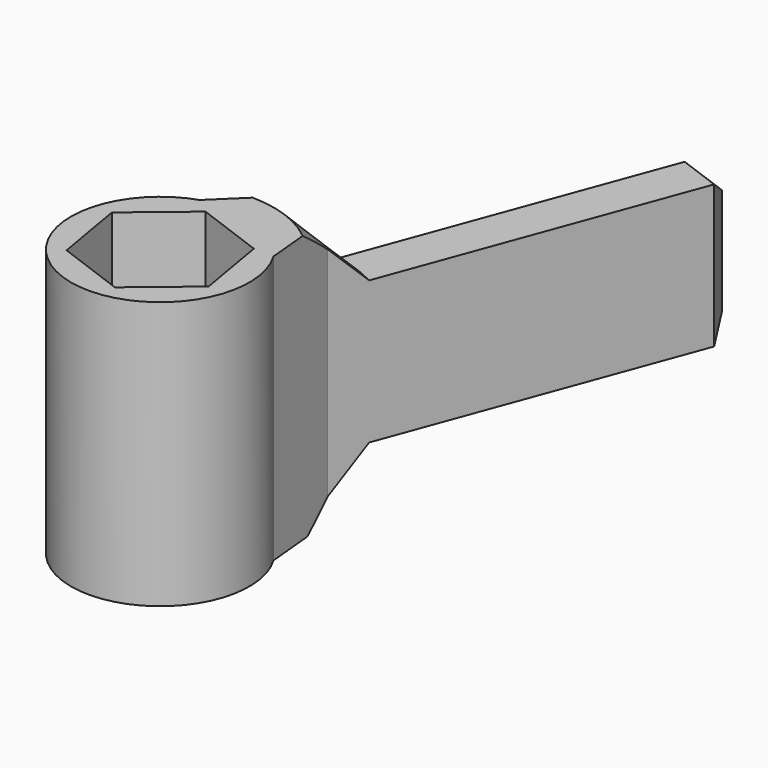
from build123d import *

# Parameters (mm, degrees)
F0_R         = 5
F1_DEPTH     = 15
F2_W         = 2.5
F2_H         = 8
F3_DEPTH     = 25
F4_T1_DEPTH  = 8
F4_T6_ANGLE  = 323.6604372277
F4_T13_ANGLE = 323.6604372277
F4_T21_ANGLE = 323.6604372277
F4_T26_DEPTH = 15.8662197745
F4_T34_ANGLE = 323.6604372277
F4_T39_DEPTH = 15.8662197745
F4_T47_DEPTH = 15.8662197745
F4_T52_ANGLE = 323.6604372277
F4_T60_ANGLE = 323.6604372277
F4_T65_DEPTH = 15.8662197745
F5_SIZE      = 1


# Not quite as in the source:
# - a fillet or chamfer that OpenCascade refuses, or shapes differently, is made with other operations: its cross-section is extruded or revolved along the edge and cut away or added


with BuildPart() as f1:
    # F0 (on Top) → F1 (new body)
    with BuildSketch(Plane.XY):
        Circle(F0_R)
        Polygon((3.1522870356, 2.6203854256), (3.8454638641, -1.4197679401), (0.6931768285, -4.0401533656), (-3.1522870356, -2.6203854256), (-3.8454638641, 1.4197679401), (-0.6931768285, 4.0401533656), align=None, mode=Mode.SUBTRACT)
    extrude(amount=F1_DEPTH)

    # F2 (on face) → F3 (join)
    with BuildSketch(Plane(origin=(1.2295551036, 3.3302693956, 0), x_dir=(0.9381040551, -0.3463535503, 0), z_dir=(-0.3463535503, -0.9381040551, 0))):
        with Locations((0, 7.3666626269)):
            Rectangle(F2_W, F2_H)
    extrude(amount=-F3_DEPTH)

    # F4: chamfer of 5 on 4 edges, made by hand

    # F4_s2 → F4_t1 (join)
    with BuildSketch(Plane.XY.offset(3.3666626269)):
        with BuildLine():
            Line((-1.5797144045, 4.7438910612), (1.5310914666, 7.7560143709))
            Line((1.5310914666, 7.7560143709), (0.5041468464, 4.9745186659))
            ThreePointArc((0.5041468464, 4.9745186659), (-0.631305898, 4.9599851676), (-1.5797144045, 4.7438910612))
        make_face()
        with BuildLine():
            Line((4.2834359399, 2.5791813718), (3.8763516043, 6.8901304951))
            Line((3.8763516043, 6.8901304951), (2.8494069841, 4.1086347901))
            ThreePointArc((2.8494069841, 4.1086347901), (3.702995808, 3.359735413), (4.2834359399, 2.5791813718))
        make_face()
    extrude(amount=F4_T1_DEPTH)


with BuildPart() as f4_tool4:
    # F4_s5 → F4_t6 (revolve)
    with BuildSketch(Plane(origin=(0, 0, 0), x_dir=(0, 0, 1), z_dir=(0.7833222839, -0.6216157974, 0))):
        Polygon((16.3666626269, 5), (11.3666626269, 10), (11.3666626269, 5), align=None)
    revolve(axis=Axis((0, 0, 11.3666626269), (0, 0, -1)), revolution_arc=F4_T6_ANGLE)

    split(bisect_by=Plane.XY.offset(15), keep=Keep.BOTTOM)

    split(bisect_by=Plane(origin=(-1.1726300689, 0.4329419379, 0), x_dir=(0, 0, 1), z_dir=(0.9381040551, -0.3463535503, 0)), keep=Keep.TOP)

    split(bisect_by=Plane(origin=(1.1726300689, -0.4329419379, 0), x_dir=(0, 0, 1), z_dir=(-0.9381040551, 0.3463535503, 0)), keep=Keep.TOP)


with BuildPart() as f1_1:
    add(f1.part)

    # F4_t3: union F4_tool4
    add(f4_tool4.part)


with BuildPart() as f4_tool11:
    # F4_s12 → F4_t13 (revolve)
    with BuildSketch(Plane(origin=(0, 0, 0), x_dir=(0, 0, 1), z_dir=(0.7833222839, -0.6216157974, 0))):
        Polygon((-1.6333373731, 5), (3.3666626269, 10), (3.3666626269, 5), align=None)
    revolve(axis=Axis((0, 0, 3.3666626269), (0, 0, -1)), revolution_arc=F4_T13_ANGLE)

    split(bisect_by=Plane.XY, keep=Keep.TOP)

    split(bisect_by=Plane(origin=(-1.1726300689, 0.4329419379, 0), x_dir=(0, 0, 1), z_dir=(0.9381040551, -0.3463535503, 0)), keep=Keep.TOP)

    split(bisect_by=Plane(origin=(1.1726300689, -0.4329419379, 0), x_dir=(0, 0, 1), z_dir=(-0.9381040551, 0.3463535503, 0)), keep=Keep.TOP)


with BuildPart() as f1_2:
    add(f1_1.part)

    # F4_t10: union F4_tool11
    add(f4_tool11.part)


with BuildPart() as f4_tool19:
    # F4_s20 → F4_t21 (revolve)
    with BuildSketch(Plane(origin=(0, 0, 0), x_dir=(0, 0, 1), z_dir=(0.7833222839, -0.6216157974, 0))):
        Polygon((16.3666626269, 5), (11.3666626269, 10), (11.3666626269, 5), align=None)
    revolve(axis=Axis((0, 0, 11.3666626269), (0, 0, -1)), revolution_arc=F4_T21_ANGLE)

    split(bisect_by=Plane.XY.offset(15), keep=Keep.BOTTOM)

    split(bisect_by=Plane(origin=(-1.1726300689, 0.4329419379, 0), x_dir=(0, 0, 1), z_dir=(-0.9381040551, 0.3463535503, 0)), keep=Keep.TOP)


with BuildPart() as f4_tool24:
    # F4_s25 → F4_t26 (new body)
    with BuildSketch(Plane.XY.offset(19.2328824014)):
        with BuildLine():
            Line((-1.5797144045, 4.7438910612), (1.5310914666, 7.7560143709))
            Line((1.5310914666, 7.7560143709), (0.5041468464, 4.9745186659))
            ThreePointArc((0.5041468464, 4.9745186659), (-0.631305898, 4.9599851676), (-1.5797144045, 4.7438910612))
        make_face()
    extrude(amount=-F4_T26_DEPTH)

    split(bisect_by=Plane.XY.offset(15), keep=Keep.BOTTOM)

    split(bisect_by=Plane.XY.offset(11.3666626269), keep=Keep.TOP)


with BuildPart() as f4_tool19_1:
    add(f4_tool19.part)

    # F4_t29: intersect F4_tool24
    add(f4_tool24.part, mode=Mode.INTERSECT)


with BuildPart() as f1_3:
    add(f1_2.part)

    # F4_t17: union F4_tool19
    add(f4_tool19_1.part)


with BuildPart() as f4_tool32:
    # F4_s33 → F4_t34 (revolve)
    with BuildSketch(Plane(origin=(0, 0, 0), x_dir=(0, 0, 1), z_dir=(0.7833222839, -0.6216157974, 0))):
        Polygon((16.3666626269, 5), (11.3666626269, 10), (11.3666626269, 5), align=None)
    revolve(axis=Axis((0, 0, 11.3666626269), (0, 0, -1)), revolution_arc=F4_T34_ANGLE)

    split(bisect_by=Plane.XY.offset(15), keep=Keep.BOTTOM)

    split(bisect_by=Plane(origin=(1.1726300689, -0.4329419379, 0), x_dir=(0, 0, 1), z_dir=(0.9381040551, -0.3463535503, 0)), keep=Keep.TOP)


with BuildPart() as f4_tool37:
    # F4_s38 → F4_t39 (new body)
    with BuildSketch(Plane.XY.offset(19.2328824014)):
        with BuildLine():
            Line((4.2834359399, 2.5791813718), (3.8763516043, 6.8901304951))
            Line((3.8763516043, 6.8901304951), (2.8494069841, 4.1086347901))
            ThreePointArc((2.8494069841, 4.1086347901), (3.702995808, 3.359735413), (4.2834359399, 2.5791813718))
        make_face()
    extrude(amount=-F4_T39_DEPTH)

    split(bisect_by=Plane.XY.offset(15), keep=Keep.BOTTOM)

    split(bisect_by=Plane.XY.offset(11.3666626269), keep=Keep.TOP)


with BuildPart() as f4_tool32_1:
    add(f4_tool32.part)

    # F4_t42: intersect F4_tool37
    add(f4_tool37.part, mode=Mode.INTERSECT)


with BuildPart() as f1_4:
    add(f1_3.part)

    # F4_t30: union F4_tool32
    add(f4_tool32_1.part)


with BuildPart() as f4_tool45:
    # F4_s46 → F4_t47 (new body)
    with BuildSketch(Plane.XY.offset(11.3666626269)):
        with BuildLine():
            Line((-1.5797144045, 4.7438910612), (1.5310914666, 7.7560143709))
            Line((1.5310914666, 7.7560143709), (0.5041468464, 4.9745186659))
            ThreePointArc((0.5041468464, 4.9745186659), (-0.631305898, 4.9599851676), (-1.5797144045, 4.7438910612))
        make_face()
    extrude(amount=-F4_T47_DEPTH)

    split(bisect_by=Plane.XY, keep=Keep.TOP)

    split(bisect_by=Plane.XY.offset(3.3666626269), keep=Keep.BOTTOM)


with BuildPart() as f4_tool50:
    # F4_s51 → F4_t52 (revolve)
    with BuildSketch(Plane(origin=(0, 0, 0), x_dir=(0, 0, 1), z_dir=(0.7833222839, -0.6216157974, 0))):
        Polygon((-1.6333373731, 5), (3.3666626269, 10), (3.3666626269, 5), align=None)
    revolve(axis=Axis((0, 0, 3.3666626269), (0, 0, -1)), revolution_arc=F4_T52_ANGLE)

    split(bisect_by=Plane.XY, keep=Keep.TOP)

    split(bisect_by=Plane(origin=(-1.1726300689, 0.4329419379, 0), x_dir=(0, 0, 1), z_dir=(-0.9381040551, 0.3463535503, 0)), keep=Keep.TOP)


with BuildPart() as f4_tool45_1:
    add(f4_tool45.part)

    # F4_t55: intersect F4_tool50
    add(f4_tool50.part, mode=Mode.INTERSECT)


with BuildPart() as f1_5:
    add(f1_4.part)

    # F4_t43: union F4_tool45
    add(f4_tool45_1.part)


with BuildPart() as f4_tool58:
    # F4_s59 → F4_t60 (revolve)
    with BuildSketch(Plane(origin=(0, 0, 0), x_dir=(0, 0, 1), z_dir=(0.7833222839, -0.6216157974, 0))):
        Polygon((-1.6333373731, 5), (3.3666626269, 10), (3.3666626269, 5), align=None)
    revolve(axis=Axis((0, 0, 3.3666626269), (0, 0, -1)), revolution_arc=F4_T60_ANGLE)

    split(bisect_by=Plane.XY, keep=Keep.TOP)

    split(bisect_by=Plane(origin=(1.1726300689, -0.4329419379, 0), x_dir=(0, 0, 1), z_dir=(0.9381040551, -0.3463535503, 0)), keep=Keep.TOP)


with BuildPart() as f4_tool63:
    # F4_s64 → F4_t65 (new body)
    with BuildSketch(Plane.XY.offset(11.3666626269)):
        with BuildLine():
            Line((4.2834359399, 2.5791813718), (3.8763516043, 6.8901304951))
            Line((3.8763516043, 6.8901304951), (2.8494069841, 4.1086347901))
            ThreePointArc((2.8494069841, 4.1086347901), (3.702995808, 3.359735413), (4.2834359399, 2.5791813718))
        make_face()
    extrude(amount=-F4_T65_DEPTH)

    split(bisect_by=Plane.XY, keep=Keep.TOP)

    split(bisect_by=Plane.XY.offset(3.3666626269), keep=Keep.BOTTOM)


with BuildPart() as f4_tool58_1:
    add(f4_tool58.part)

    # F4_t68: intersect F4_tool63
    add(f4_tool63.part, mode=Mode.INTERSECT)


with BuildPart() as f1_6:
    add(f1_5.part)

    # F4_t56: union F4_tool58
    add(f4_tool58_1.part)

    # F5
    f5_edges = [f1_6.edges().sort_by_distance(p)[0] for p in [
        (11.061024, 26.349929, 7.366663),
        (9.888394, 26.782871, 11.366663),
        (8.715764, 27.215813, 7.366663),
        (9.888394, 26.782871, 3.366663),
    ]]
    chamfer(f5_edges, length=F5_SIZE)


solid = f1_6.part
